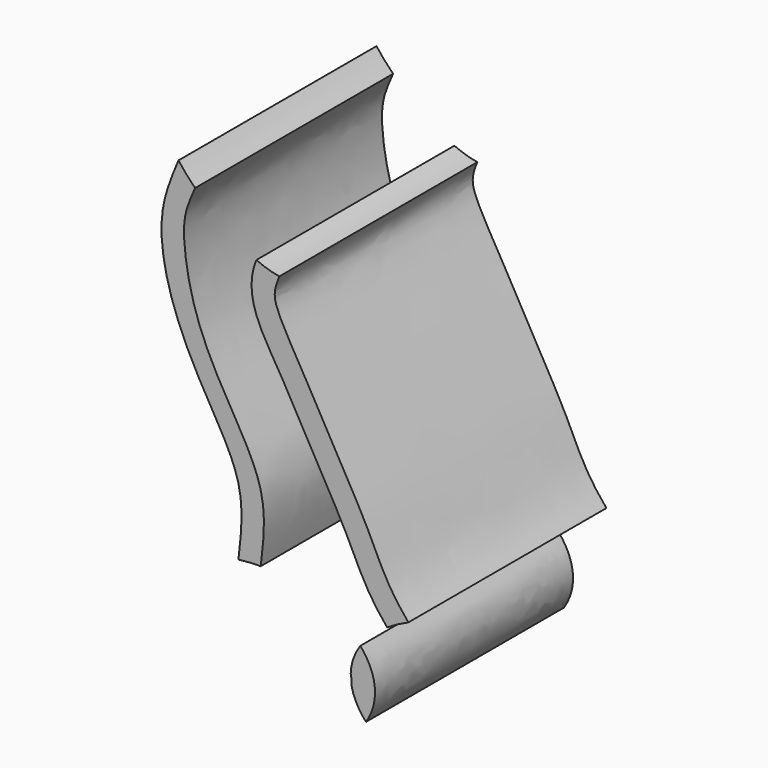
from build123d import *

# Parameters (mm, degrees)
F1_DEPTH = 50.8


# Not quite as in the source:
# - a feature names something its author has since deleted; it is built from what else it names


with BuildPart() as f1:
    # F0 (on Front) → F1 (new body)
    with BuildSketch(Plane.XZ):
        with BuildLine():
            add(Edge.make_bspline(
                [(-24.3141159331, 26.1021399349), (-26.6260970552, 26.1057942616), (-28.8948994559, 25.8185440872)],
                knots=[1.5683489444, 1.5683489444, 1.5683489444, 1.7643806816, 1.7643806816, 1.7643806816], degree=2, weights=[1, 0.9952002892, 1]))
            add(Edge.make_bspline(
                [(-24.3141159331, 26.1021399349), (-23.7504685709, 30.7816022131), (-22.6573335885, 39.7966807836), (-31.0371752335, 53.456246822), (-38.5489160591, 67.3127661846), (-40.9073074567, 83.4789578935), (-38.987254402, 87.2492337999), (-37.7880842583, 90.0557118677)],
                knots=[0, 0, 0, 0, 0.2002565357, 0.4141172276, 0.6374458564, 0.8497473054, 0.9956221455, 0.9956221455, 0.9956221455, 0.9956221455], degree=3))
            add(Edge.make_bspline(
                [(-41.1941618229, 93.9520463131), (-40.2207372717, 92.6374220537), (-39.0620502408, 91.3242148197), (-37.7880842583, 90.0557118677)],
                knots=[0.1145347036, 0.1145347036, 0.1145347036, 0.1145347036, 0.1557606283, 0.1557606283, 0.1557606283, 0.1557606283], degree=3))
            add(Edge.make_bspline(
                [(-28.8948994559, 25.8185440872), (-28.3516476874, 30.3286799071), (-27.2234114209, 39.6269273648), (-35.638432395, 53.0342333907), (-43.0621524761, 67.4698179733), (-45.8697930663, 82.837401957), (-42.6908916889, 90.4240239555), (-41.1941618229, 93.9520463131)],
                knots=[0, 0, 0, 0, 0.193010248, 0.3991323855, 0.6143798623, 0.8189991781, 0.997394633, 0.997394633, 0.997394633, 0.997394633], degree=3))
        make_face()
    extrude(amount=F1_DEPTH)


with BuildPart() as f1b:
    # F0 (on Front) → F1, piece 2 (new body)
    with BuildSketch(Plane.XZ):
        with BuildLine():
            add(Edge.make_bspline(
                [(-0.8593497944, 10.9171546791), (-0.8593497944, 14.8987735909), (-3.884425209, 18.3681205211)],
                knots=[0, 0, 0, 0.5128680966, 0.5128680966, 0.5128680966], degree=2, weights=[1, 0.9673005687, 1]))
            add(Edge.make_bspline(
                [(-3.884425209, 18.3681205211), (-5.7694255428, 15.6159078961), (-5.8530664589, 12.6887294195)],
                knots=[2.7937773438, 2.7937773438, 2.7937773438, 3.1264681713, 3.1264681713, 3.1264681713], degree=2, weights=[1, 0.9861964753, 1]))
            add(Edge.make_bspline(
                [(-5.6510078625, 10.9171546791), (-5.6510078625, 11.8077482948), (-5.8530664589, 12.6887294195)],
                knots=[0, 0, 0, 0.147056621, 0.147056621, 0.147056621], degree=2, weights=[1, 0.9972980114, 1]))
            add(Edge.make_bspline(
                [(-5.6608244172, 10.5256666684), (-5.6510078625, 10.7213593391), (-5.6510078625, 10.9171546791)],
                knots=[6.2507996255, 6.2507996255, 6.2507996255, 6.2831853072, 6.2831853072, 6.2831853072], degree=2, weights=[1, 0.9998688988, 1]))
            add(Edge.make_bspline(
                [(-5.6608244172, 10.5256666684), (-5.0617599039, 7.6318214617), (-2.7192334462, 4.9979547786)],
                knots=[3.2507399401, 3.2507399401, 3.2507399401, 3.5816071025, 3.5816071025, 3.5816071025], degree=2, weights=[1, 0.9863470459, 1]))
            add(Edge.make_bspline(
                [(-2.7192334462, 4.9979547786), (-0.8593497944, 7.8356784138), (-0.8593497944, 10.9171546791)],
                knots=[5.8827655458, 5.8827655458, 5.8827655458, 6.2831853072, 6.2831853072, 6.2831853072], degree=2, weights=[1, 0.9800248594, 1]))
        make_face()
    extrude(amount=F1_DEPTH)


with BuildPart() as f1c:
    # F0 (on Front) → F1, piece 3 (new body)
    with BuildSketch(Plane.XZ):
        with BuildLine():
            add(Edge.make_bspline(
                [(1.6275324331, 23.4913965441), (-2.5781939039, 28.3605122499), (-5.7531419947, 36.5388547463), (-13.843696099, 50.3742483725), (-20.181170777, 62.2846491187), (-26.1336358697, 71.3016463879), (-26.6173623264, 77.7683902544), (-25.2118867969, 81.1500811666)],
                knots=[0, 0, 0, 0, 0.2201847678, 0.4398977895, 0.6466164756, 0.82714544, 0.9983698701, 0.9983698701, 0.9983698701, 0.9983698701], degree=3))
            add(Edge.make_bspline(
                [(5.9918386386, 25.8185440664), (3.6020725269, 24.7640726232), (1.6275324331, 23.4913965441)],
                knots=[2.2656666605, 2.2656666605, 2.2656666605, 2.4540091157, 2.4540091157, 2.4540091157], degree=2, weights=[1, 0.9955691659, 1]))
            add(Edge.make_bspline(
                [(5.9918386386, 25.8185440664), (1.6159325214, 30.8846828247), (-1.3008960748, 38.7397948712), (-9.5296098113, 52.8425702091), (-15.7126231247, 64.2182177816), (-21.6591543897, 74.1423833807), (-21.6600143389, 76.9665087767), (-20.4903893837, 79.7229993409)],
                knots=[0, 0, 0, 0, 0.229094286, 0.4576977372, 0.6727810523, 0.8606149094, 1, 1, 1, 1], degree=3))
            add(Edge.make_bspline(
                [(-25.2118867969, 81.1500811666), (-23.5876635098, 80.4401666232), (-21.9982141694, 79.9443299939), (-20.4903893837, 79.7229993409)],
                knots=[0.2764650159, 0.2764650159, 0.2764650159, 0.2764650159, 0.3225195587, 0.3225195587, 0.3225195587, 0.3225195587], degree=3))
        make_face()
    extrude(amount=F1_DEPTH)


solid = Compound([f1.part, f1b.part, f1c.part])
